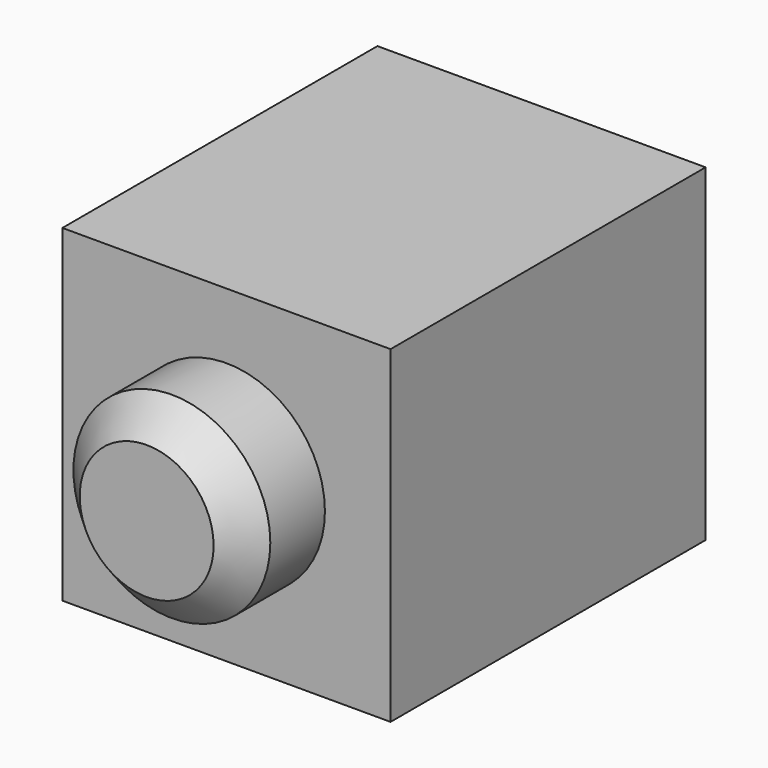
from build123d import *

# Parameters (mm, degrees)
F0_W     = 15.875
F0_H     = 15.875
F1_DEPTH = 19.05
F2_R     = 4.7625
F3_DEPTH = 4.826
F4_SIZE  = 1.524
F5_T     = -1.5875


with BuildPart() as f1:
    # F0 (on Front) → F1 (new body)
    with BuildSketch(Plane.XZ):
        Rectangle(F0_W, F0_H)
    extrude(amount=F1_DEPTH)

    # F2 (on face) → F3 (join)
    with BuildSketch(Plane.XZ.offset(19.05)):
        Circle(F2_R)
    extrude(amount=F3_DEPTH)

    # F4
    f4_edges = [f1.edges().sort_by_distance(p)[0] for p in [
        (-4.7625, -23.876, 0),
    ]]
    chamfer(f4_edges, length=F4_SIZE)

    # F5
    f5_openings = [f1.faces().sort_by_distance(p)[0] for p in [
        (0, 0, 0),
    ]]
    offset(amount=F5_T, openings=f5_openings, kind=Kind.INTERSECTION)


solid = f1.part
